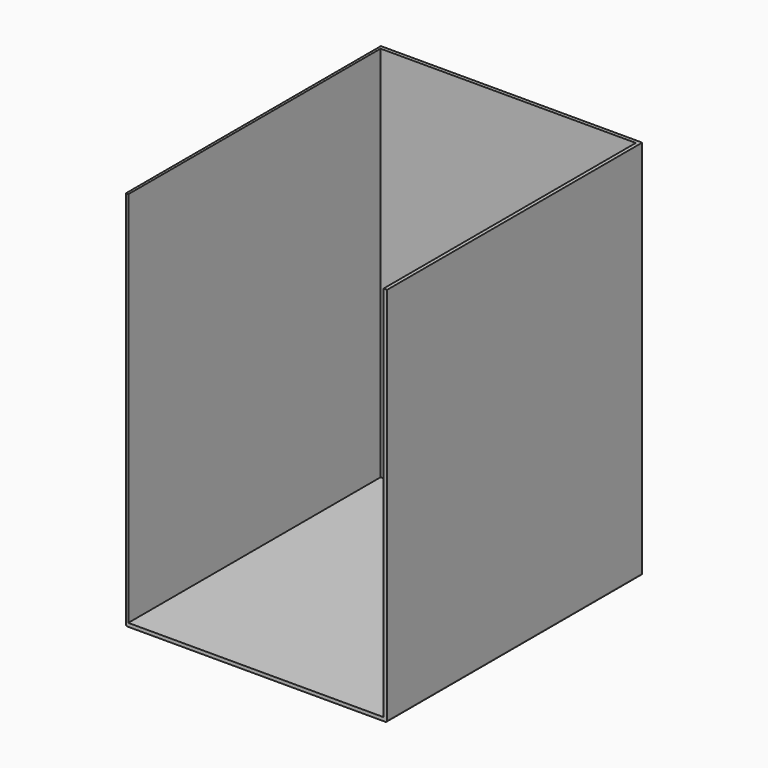
from build123d import *

# Parameters (mm, degrees)
F1_DEPTH = 426
F2_W     = 295
F2_H     = 360
F3_DEPTH = 4
F4_R     = 2


# Not quite as in the source:
# - a feature names something its author has since deleted; it is built from what else it names


with BuildPart() as f1:
    # F0 (on Top) → F1 (new body)
    with BuildSketch(Plane.XY):
        Polygon((-4, -360), (0, -360), (0, 0), (-295, 0), (-295, -360), (-292.1838745495, -360), (-292.1838745495, -4), (-4, -4), align=None)
    extrude(amount=F1_DEPTH)

    # F2 (on Top) → F3 (join)
    with BuildSketch(Plane.XY):
        with Locations((-147.5, -180)):
            Rectangle(F2_W, F2_H)
    extrude(amount=-F3_DEPTH)

    # F4
    f4_edges = [f1.edges().sort_by_distance(p)[0] for p in [
        (-295, -180, -4),
        (0, -180, -4),
    ]]
    fillet(f4_edges, radius=F4_R)


solid = f1.part
